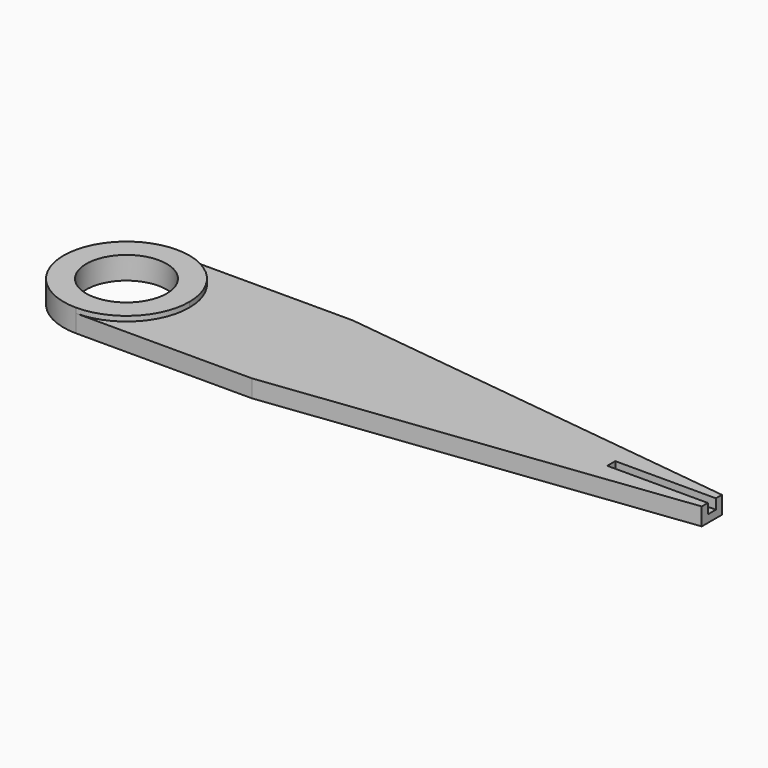
from build123d import *

# Parameters (mm, degrees)
F0_R         = 8
F1_DEPTH     = 3.5
F2_R         = 8
F3_DEPTH     = 1
F4_W         = 20
F4_H         = 2
F5_DEPTH     = 2
F6_TEXT_SIZE = 18.6788435611
F7_DEPTH     = 1


# Not quite as in the source:
# - Text() gives the source's letters only with a copy of the font that has no kerning and outlines rounded to 1/6400 em; it was checked with that copy


with BuildPart() as f1:
    # F0 (on Top) → F1 (new body)
    with BuildSketch(Plane.XY):
        with BuildLine():
            ThreePointArc((0, -12.5), (8.8388347648, -8.8388347648), (12.5, 0))
            ThreePointArc((12.5, 0), (8.8388347648, 8.8388347648), (0, 12.5))
            ThreePointArc((0, 12.5), (-12.5, 0), (0, -12.5))
        make_face()
        Circle(F0_R, mode=Mode.SUBTRACT)
        with BuildLine():
            ThreePointArc((0, 12.5), (8.8388347648, 8.8388347648), (12.5, 0))
            ThreePointArc((12.5, 0), (8.8388347648, -8.8388347648), (0, -12.5))
            Line((0, -12.5), (35, -12.5))
            Line((35, -12.5), (116.3887844346, -2.5067138408))
            Line((116.3887844346, -2.5067138408), (116.3887844346, 2.5067138408))
            Line((116.3887844346, 2.5067138408), (35, 12.5))
            Line((35, 12.5), (0, 12.5))
        make_face()
    extrude(amount=F1_DEPTH)

    # F2 (on face) → F3 (join)
    with BuildSketch(Plane.XY.offset(3.5)):
        with BuildLine():
            ThreePointArc((0, -12.5), (8.8388347648, -8.8388347648), (12.5, 0))
            ThreePointArc((12.5, 0), (8.8388347648, 8.8388347648), (0, 12.5))
            ThreePointArc((0, 12.5), (-12.5, 0), (0, -12.5))
        make_face()
        Circle(F2_R, mode=Mode.SUBTRACT)
    extrude(amount=F3_DEPTH)

    # F4 (on face) → F5 (cut)
    with BuildSketch(Plane.XY.offset(3.5)):
        with Locations((106.3887844346, 0.0067138408)):
            Rectangle(F4_W, F4_H)
    extrude(amount=-F5_DEPTH, mode=Mode.SUBTRACT)

    # F6 (on face) → F7 (join)
    with BuildSketch(Plane(origin=(0, 0, 0), x_dir=(1, 0, 0), z_dir=(0, 0, -1))):
        with Locations((17.4069125205, -7.0232450962)):
            Text('SEAN', F6_TEXT_SIZE, font='Open Sans', text_align=(TextAlign.LEFT, TextAlign.BOTTOM))
    extrude(amount=F7_DEPTH)


solid = f1.part
